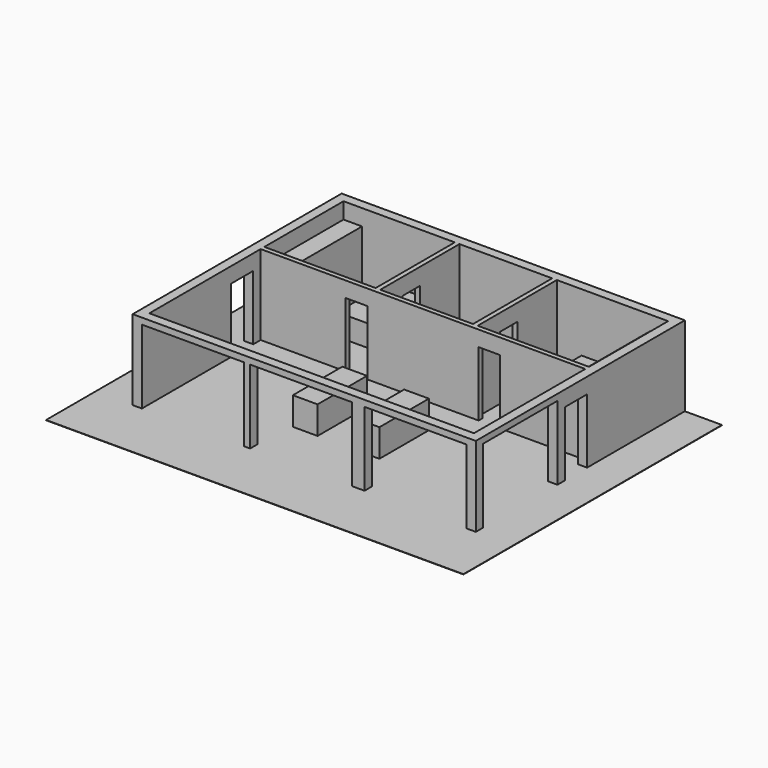
from build123d import *

# Parameters (mm, degrees)
F0_W      = 11100
F0_H      = 8450
F0_W_2    = 10500
F0_H_2    = 4500
F0_W_3    = 3600
F0_H_3    = 3200
F0_W_4    = 3000
F1_DEPTH  = 2600
F2_W      = 700
F2_H      = 2100
F3_DEPTH  = 150
F4_W      = 900
F4_H      = 2100
F5_DEPTH  = 300
F6_W      = 900
F6_H      = 2100
F7_DEPTH  = 300
F8_W      = 3000
F8_H      = 2400
F10_DEPTH = 300
F11_W     = 3300
F11_H     = 2400
F12_DEPTH = 300
F13_W     = 13500
F13_H     = 10450
F14_DEPTH = 10
F15_W     = 3200
F15_H     = 2068.0467987061
F16_DEPTH = 600
F17_W     = 3200
F17_H     = 2100
F18_DEPTH = 600
F19_W     = 3000
F19_H     = 2049.3771934509
F20_DEPTH = 600
F21_W     = 1400
F21_H     = 2000
F22_DEPTH = 700
F23_W     = 1400
F23_H     = 2000
F24_DEPTH = 700
F25_W     = 700
F25_H     = 2049.3771934509
F26_DEPTH = 150
F27_W     = 700
F27_H     = 2049.3771934509
F28_DEPTH = 150
F29_W     = 800
F29_H     = 2000
F30_DEPTH = 900


# Not quite as in the source:
# - a feature names something its author has since deleted; it is built from what else it names


with BuildPart() as f1:
    # F0 (on Top) → F1 (new body)
    with BuildSketch(Plane.XY):
        with Locations((5250, -725)):
            Rectangle(F0_W, F0_H)
        with Locations((5250, -2400)):
            Rectangle(F0_W_2, F0_H_2, mode=Mode.SUBTRACT)
        with Locations((1800, 1600)):
            Rectangle(F0_W_3, F0_H_3, mode=Mode.SUBTRACT)
        with Locations((5250, 1600)):
            Rectangle(F0_W_4, F0_H_3, mode=Mode.SUBTRACT)
        with Locations((8700, 1600)):
            Rectangle(F0_W_3, F0_H_3, mode=Mode.SUBTRACT)
    extrude(amount=F1_DEPTH)

    # F2 (on face) → F3 (cut, through all)
    with BuildSketch(Plane(origin=(0, 0, 0), x_dir=(-1, 0, 0), z_dir=(0, 1, 0))):
        with Locations((-7400, 1050)):
            Rectangle(F2_W, F2_H)
        with Locations((-3100, 1050)):
            Rectangle(F2_W, F2_H)
    extrude(amount=-F3_DEPTH, mode=Mode.SUBTRACT)

    # F4 (on face) → F5 (cut, through all)
    with BuildSketch(Plane(origin=(10500, 0, 0), x_dir=(0, -1, 0), z_dir=(-1, 0, 0))):
        with Locations((900, 1050)):
            Rectangle(F4_W, F4_H)
    extrude(amount=-F5_DEPTH, mode=Mode.SUBTRACT)

    # F6 (on face) → F7 (cut, through all)
    with BuildSketch(Plane.YZ):
        with Locations((-900, 1050)):
            Rectangle(F6_W, F6_H)
    extrude(amount=-F7_DEPTH, mode=Mode.SUBTRACT)

    # F8 (on face) → F10 (cut, through all)
    with BuildSketch(Plane(origin=(10500, 0, 0), x_dir=(0, -1, 0), z_dir=(-1, 0, 0))):
        with Locations((3150, 1200)):
            Rectangle(F8_W, F8_H)
    extrude(amount=-F10_DEPTH, mode=Mode.SUBTRACT)

    # F11 (on face) → F12 (cut, through all)
    with BuildSketch(Plane(origin=(0, -4650, 0), x_dir=(-1, 0, 0), z_dir=(0, 1, 0))):
        with Locations((-8850, 1200)):
            Rectangle(F11_W, F11_H)
        with Locations((-5150, 1200)):
            Rectangle(F11_W, F11_H)
        with Locations((-1650, 1200)):
            Rectangle(F11_W, F11_H)
    extrude(amount=-F12_DEPTH, mode=Mode.SUBTRACT)

    # F13 (on Top) → F14 (join)
    with BuildSketch(Plane.XY):
        with Locations((5250, -1725)):
            Rectangle(F13_W, F13_H)
    extrude(amount=F14_DEPTH)

    # F15 (on face) → F16 (join)
    with BuildSketch(Plane.YZ):
        with Locations((1600, 1044.023399353)):
            Rectangle(F15_W, F15_H)
    extrude(amount=F16_DEPTH)

    # F17 (on face) → F18 (join)
    with BuildSketch(Plane(origin=(10500, 0, 0), x_dir=(0, -1, 0), z_dir=(-1, 0, 0))):
        with Locations((-1600, 1060)):
            Rectangle(F17_W, F17_H)
    extrude(amount=F18_DEPTH)

    # F19 (on face) → F20 (join)
    with BuildSketch(Plane(origin=(0, 0, 0), x_dir=(-1, 0, 0), z_dir=(0, 1, 0))):
        with Locations((-5250, 1034.6885967255)):
            Rectangle(F19_W, F19_H)
    extrude(amount=F20_DEPTH)

    # F21 (on face) → F22 (join)
    with BuildSketch(Plane.XY.offset(10)):
        with Locations((2100, 2200)):
            Rectangle(F21_W, F21_H)
    extrude(amount=F22_DEPTH)

    # F23 (on face) → F24 (join)
    with BuildSketch(Plane.XY.offset(10)):
        with Locations((8400, 2200)):
            Rectangle(F23_W, F23_H)
    extrude(amount=F24_DEPTH)

    # F25 (on face) → F26 (cut, through all)
    with BuildSketch(Plane(origin=(6750, 0, 0), x_dir=(0, -1, 0), z_dir=(-1, 0, 0))):
        with Locations((-1250, 1034.6885967255)):
            Rectangle(F25_W, F25_H)
    extrude(amount=-F26_DEPTH, mode=Mode.SUBTRACT)

    # F27 (on face) → F28 (cut, through all)
    with BuildSketch(Plane.YZ.offset(3750)):
        with Locations((1250, 1034.6885967255)):
            Rectangle(F27_W, F27_H)
    extrude(amount=-F28_DEPTH, mode=Mode.SUBTRACT)

    # F29 (on face) → F30 (join)
    with BuildSketch(Plane.XY.offset(10)):
        with Locations((4001.805305481, -2350)):
            Rectangle(F29_W, F29_H)
        with Locations((6001.805305481, -2350)):
            Rectangle(F29_W, F29_H)
    extrude(amount=F30_DEPTH)


solid = f1.part
